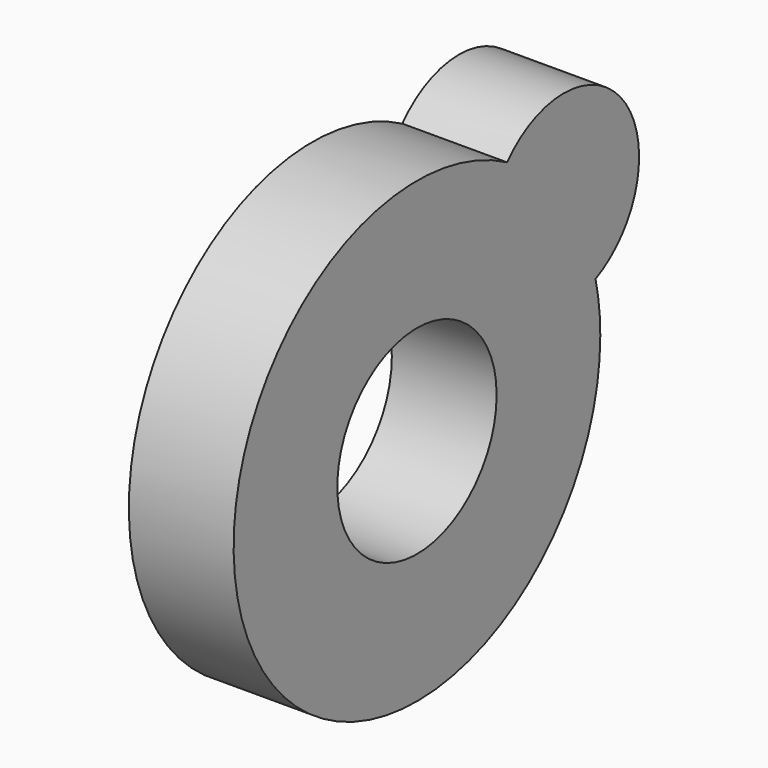
from build123d import *

# Parameters (mm, degrees)
F1_DEPTH = 25.4
F3_R     = 24.1381170573
F4_DEPTH = 25.4


# Not quite as in the source:
# - the program builds the solid bodies; features that only make, move or delete a surface that nothing else refers to are left out


with BuildPart() as f1:
    # F0 (on Right) → F1 (new body)
    with BuildSketch(Plane.YZ):
        with BuildLine():
            ThreePointArc((27.3132670653, 48.3872874563), (-47.984242661, -28.0152922777), (55.5638744614, 0))
            ThreePointArc((55.5638744614, 0), (55.2010789182, 6.3391664614), (54.1174299211, 12.5955517503))
            ThreePointArc((54.1174299211, 12.5955517503), (26.1882593397, 19.6121913174), (27.3132670653, 48.3872874563))
        make_face()
        with BuildLine():
            ThreePointArc((27.3132670653, 48.3872874563), (26.1882593397, 19.6121913174), (54.1174299211, 12.5955517503))
            ThreePointArc((54.1174299211, 12.5955517503), (44.4747309057, 33.3067929411), (27.3132670653, 48.3872874563))
        make_face()
        with BuildLine():
            ThreePointArc((27.3132670653, 48.3872874563), (44.4747309057, 33.3067929411), (54.1174299211, 12.5955517503))
            ThreePointArc((54.1174299211, 12.5955517503), (63.739124452, 21.0259013912), (67.3206748777, 33.3067929411))
            ThreePointArc((67.3206748777, 33.3067929411), (52.5328732039, 54.6844330979), (27.3132670653, 48.3872874563))
        make_face()
    extrude(amount=F1_DEPTH)

    # F3 (on face) → F4 (cut)
    with BuildSketch(Plane.YZ.offset(25.4)):
        Circle(F3_R)
    extrude(amount=-F4_DEPTH, mode=Mode.SUBTRACT)


solid = f1.part
